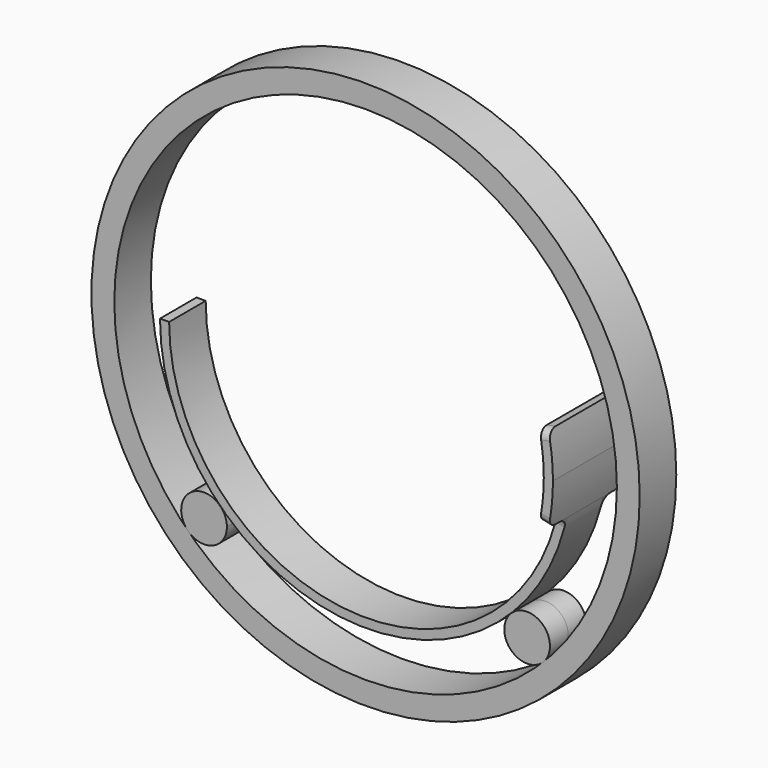
from build123d import *

# Parameters (mm, degrees)
F1_R         = 76.2
F2_DEPTH     = 6.35
F5_DEPTH     = 6.35
F6_DEPTH     = 12.7
F7_T4_DEPTH  = 15.24
F7_S5_R      = 54.61
F7_T6_DEPTH  = 10
F7_S7_R      = 57.15
F7_T8_DEPTH  = 10
F7_T12_DEPTH = 15.24
F7_S13_R     = 54.61
F7_T14_DEPTH = 10
F7_S15_R     = 57.15
F7_T16_DEPTH = 10
F7_T17_DEPTH = 15.24
F7_T19_DEPTH = 15.24


# Not quite as in the source:
# - a fillet or chamfer that OpenCascade refuses, or shapes differently, is made with other operations: its cross-section is extruded or revolved along the edge and cut away or added
# - a feature of the source that left no trace in its solid (it failed there, or was rolled back) is left out
# - a pattern or mirror of a feature is missing from the dataset's text; its kind, count and spacing are read off the source's solid


with BuildPart() as f2:
    # F1 (on Front) → F2 (new body, symmetric)
    with BuildSketch(Plane.XZ):
        Circle(F1_R)
        with BuildLine():
            ThreePointArc((-49.3914086403, -49.3914086914), (-26.7304377674, 64.532985339), (69.85, 0))
            ThreePointArc((69.85, 0), (26.7304377674, -64.532985339), (-49.3914086403, -49.3914086914))
        make_face(mode=Mode.SUBTRACT)
    extrude(amount=F2_DEPTH, both=True)


with BuildPart() as f2b:
    # F1 (on Front) → F2, piece 2 (new body, symmetric)
    with BuildSketch(Plane.XZ):
        with BuildLine():
            ThreePointArc((-38.5512806053, -44.9012806053), (-47.3313204176, -39.0346455808), (-49.3914086403, -49.3914086914))
            ThreePointArc((-49.3914086403, -49.3914086914), (-42.4712407931, -50.7679156299), (-38.5512806053, -44.9012806053))
        make_face()
    extrude(amount=F2_DEPTH, both=True)


with BuildPart() as f2_2_copies_1:
    # F2_2_copies: instance of F2b
    add(f2b.part.mirror(Plane(origin=(0, 0, 0), x_dir=(0, 0, 1), z_dir=(1, 0, 0))))


with BuildPart() as f5:
    # F4 (on Front) → F5 (new body, symmetric)
    with BuildSketch(Plane.XZ):
        with BuildLine():
            ThreePointArc((-57.15, 0), (-6.0275497336, -56.831251475), (55.8785614771, -11.9878633311))
            Line((55.8785614771, -11.9878633311), (53.3950698559, -11.4550694053))
            ThreePointArc((53.3950698559, -11.4550694053), (-5.7596586343, -54.3054180761), (-54.61, 0))
            Line((-54.61, 0), (-57.15, 0))
        make_face()
    extrude(amount=F5_DEPTH, both=True)

    # F4 (on Front) → F6 (join, symmetric)
    with BuildSketch(Plane.XZ):
        with BuildLine():
            Line((54.61, 0), (57.15, 0))
            ThreePointArc((57.15, 0), (56.831251475, 6.0275497336), (55.8785614771, 11.9878633311))
            Line((55.8785614771, 11.9878633311), (53.3950698559, 11.4550694053))
            ThreePointArc((53.3950698559, 11.4550694053), (54.3054180761, 5.7596586343), (54.61, 0))
        make_face()
        with BuildLine():
            ThreePointArc((55.8785614771, -11.9878633311), (56.831251475, -6.0275497336), (57.15, 0))
            Line((57.15, 0), (54.61, 0))
            ThreePointArc((54.61, 0), (54.3054180761, -5.7596586343), (53.3950698559, -11.4550694053))
            Line((53.3950698559, -11.4550694053), (55.8785614771, -11.9878633311))
        make_face()
    extrude(amount=F6_DEPTH, both=True)

    # F7: fillet of radius 2.54 on 6 edges, made by hand


with BuildPart() as f7_tool2:
    # F7_s3 → F7_t4 (new body)
    with BuildSketch(Plane(origin=(62.0872905302, 0, -13.3198481457), x_dir=(0, 1, 0), z_dir=(-0.9777526068, 0, 0.2097613881))):
        with BuildLine():
            ThreePointArc((8.89, 0), (7.0939487758, 0.7439487758), (6.35, 2.54))
            Line((6.35, 2.54), (6.35, 0))
            Line((6.35, 0), (8.89, 0))
        make_face()
    extrude(amount=F7_T4_DEPTH)

    # F7_s5 → F7_t6 (cut, symmetric)
    with BuildSketch(Plane.XZ.offset(-7.6)):
        Circle(F7_S5_R)
    extrude(amount=F7_T6_DEPTH, both=True, mode=Mode.SUBTRACT)

    # F7_s7 → F7_t8 (intersect, symmetric)
    with BuildSketch(Plane.XZ.offset(-7.6)):
        Circle(F7_S7_R)
    extrude(amount=F7_T8_DEPTH, both=True, mode=Mode.INTERSECT)


with BuildPart() as f5_1:
    add(f5.part)

    # F7_t1: union F7_tool2
    add(f7_tool2.part)


with BuildPart() as f7_tool10:
    # F7_s11 → F7_t12 (new body)
    with BuildSketch(Plane(origin=(62.0872905302, 0, -13.3198481457), x_dir=(0, 1, 0), z_dir=(-0.9777526068, 0, 0.2097613881))):
        with BuildLine():
            ThreePointArc((-8.89, 0), (-7.0939487758, 0.7439487758), (-6.35, 2.54))
            Line((-6.35, 2.54), (-6.35, 0))
            Line((-6.35, 0), (-8.89, 0))
        make_face()
    extrude(amount=F7_T12_DEPTH)

    # F7_s13 → F7_t14 (cut, symmetric)
    with BuildSketch(Plane.XZ.offset(7.6)):
        Circle(F7_S13_R)
    extrude(amount=F7_T14_DEPTH, both=True, mode=Mode.SUBTRACT)

    # F7_s15 → F7_t16 (intersect, symmetric)
    with BuildSketch(Plane.XZ.offset(7.6)):
        Circle(F7_S15_R)
    extrude(amount=F7_T16_DEPTH, both=True, mode=Mode.INTERSECT)


with BuildPart() as f5_2:
    add(f5_1.part)

    # F7_t9: union F7_tool10
    add(f7_tool10.part)

    # F7_s18 → F7_t17 (cut)
    with BuildSketch(Plane(origin=(47.1863408029, 0, -10.1230845907), x_dir=(0, 1, 0), z_dir=(0.9777526068, 0, -0.2097613881))):
        with BuildLine():
            ThreePointArc((-10.16, 0), (-11.9560512242, 0.7439487758), (-12.7, 2.54))
            Line((-12.7, 2.54), (-12.7, 0))
            Line((-12.7, 0), (-10.16, 0))
        make_face()
        with BuildLine():
            ThreePointArc((12.7, 2.54), (11.9560512242, 0.7439487758), (10.16, 0))
            Line((10.16, 0), (12.7, 0))
            Line((12.7, 0), (12.7, 2.54))
        make_face()
    extrude(amount=F7_T17_DEPTH, mode=Mode.SUBTRACT)

    # F7_s20 → F7_t19 (cut)
    with BuildSketch(Plane(origin=(62.0872905302, 0, 13.3198481457), x_dir=(0, 1, 0), z_dir=(-0.9777526068, 0, -0.2097613881))):
        with BuildLine():
            ThreePointArc((-12.7, 2.54), (-11.9560512242, 0.7439487758), (-10.16, 0))
            Line((-10.16, 0), (-12.7, 0))
            Line((-12.7, 0), (-12.7, 2.54))
        make_face()
        with BuildLine():
            ThreePointArc((12.7, 2.54), (11.9560512242, 0.7439487758), (10.16, 0))
            Line((10.16, 0), (12.7, 0))
            Line((12.7, 0), (12.7, 2.54))
        make_face()
    extrude(amount=F7_T19_DEPTH, mode=Mode.SUBTRACT)


solid = Compound([f2.part, f2b.part, f2_2_copies_1.part, f5_2.part])
